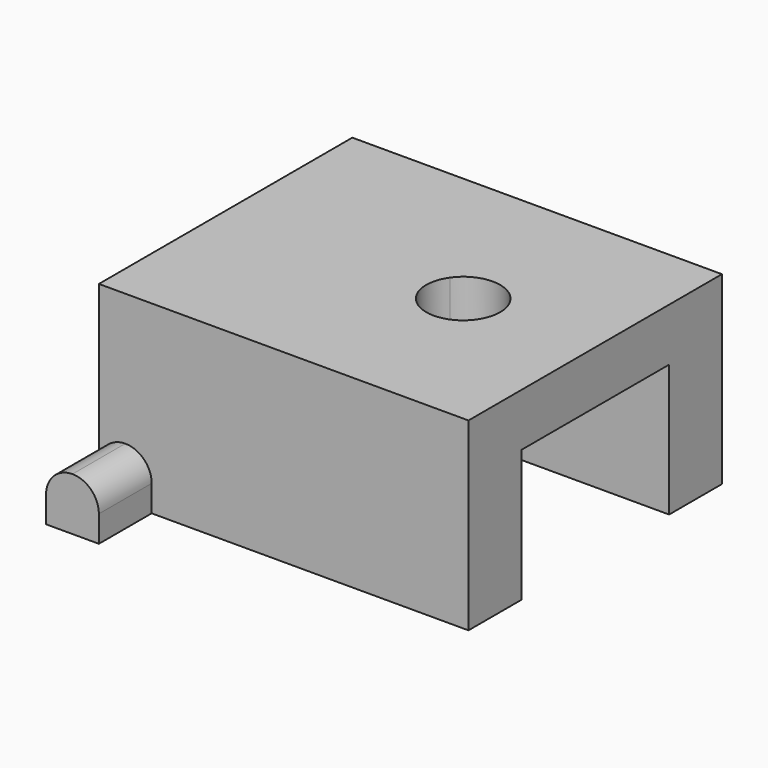
from build123d import *

# Parameters (mm, degrees)
F0_W          = 2.54
F0_H          = 2.54
F1_DEPTH      = 21.59
F3_DEPTH      = 2.54
F3_DEPTH_BACK = 2.54
F5_DEPTH      = 12.7
F7_DEPTH      = 25.4
F8_R          = 1.26999


# Not quite as in the source:
# - a fillet or chamfer is up to 0.001 mm smaller than in the source, because OpenCascade refuses the exact size


with BuildPart() as f1:
    # F0 (on Front) → F1 (new body)
    with BuildSketch(Plane.XZ):
        with Locations((1.27, 1.27)):
            Rectangle(F0_W, F0_H)
    extrude(amount=F1_DEPTH)

    # F2 (on face) → F3 (join, two sides)
    with BuildSketch(Plane.YZ.offset(2.54)) as f3_sk:
        Polygon((-18.415, 8.89), (-18.415, 2.54), (-18.415, 0), (-3.175, 0), (-3.175, 2.54), (-3.175, 8.89), align=None)
    extrude(amount=F3_DEPTH)
    extrude(f3_sk.sketch, amount=-F3_DEPTH_BACK)

    # F4 (on face) → F5 (join)
    with BuildSketch(Plane.YZ.offset(5.08)):
        Polygon((-18.415, 8.89), (-18.415, 0), (-15.24, 0), (-15.24, 6.35), (-6.35, 6.35), (-6.35, 0), (-3.175, 0), (-3.175, 8.89), align=None)
    extrude(amount=F5_DEPTH)

    # F6 (on face) → F7 (cut)
    with BuildSketch(Plane(origin=(0, 0, 6.35), x_dir=(1, 0, 0), z_dir=(0, 0, -1))):
        with BuildLine():
            ThreePointArc((12.8865943547, 11.8146160483), (10.4103839517, 12.2515943547), (9.9734056453, 9.7753839517))
            Line((9.9734056453, 9.7753839517), (12.8865943547, 11.8146160483))
        make_face()
        with BuildLine():
            Line((12.8865943547, 11.8146160483), (9.9734056453, 9.7753839517))
            ThreePointArc((9.9734056453, 9.7753839517), (11.9645368263, 9.099254034), (13.208, 10.795))
            ThreePointArc((13.208, 10.795), (13.125745966, 11.3295368263), (12.8865943547, 11.8146160483))
        make_face()
    extrude(amount=-F7_DEPTH, mode=Mode.SUBTRACT)

    # F8 (radius 1.27 in the source; OpenCascade refuses exactly that, so slightly less here)
    f8_edges = [f1.edges().sort_by_distance(p)[0] for p in [
        (0, -1.5875, 2.54),
        (2.54, -1.5875, 2.54),
        (0, -20.0025, 2.54),
        (2.54, -20.0025, 2.54),
    ]]
    fillet(f8_edges, radius=F8_R)


solid = f1.part
